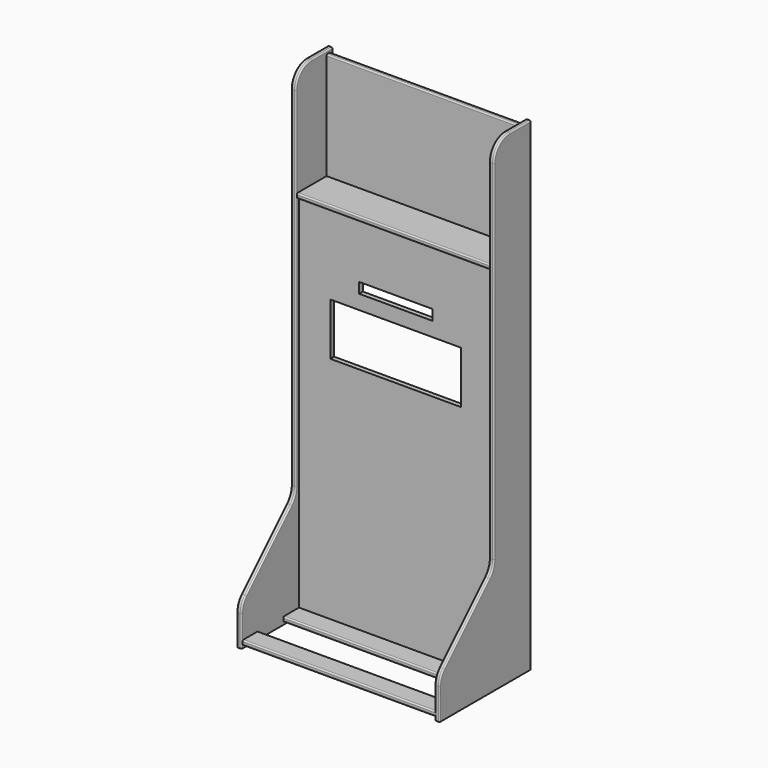
from build123d import *

# Parameters (mm, degrees)
F1_DEPTH  = 18
F3_W      = 740
F3_H      = 1382
F3_W_2    = 500
F3_H_2    = 200
F3_W_3    = 280
F3_H_3    = 40
F4_DEPTH  = 18
F7_DEPTH  = 18
F9_W      = 740
F9_H      = 160
F10_DEPTH = 18
F12_W     = 740
F12_H     = 410
F13_DEPTH = 18
F15_W     = 740
F15_H     = 225
F15_H_2   = 75
F16_DEPTH = 18
F17_R     = 4.9999


# Not quite as in the source:
# - a fillet or chamfer is up to 0.001 mm smaller than in the source, because OpenCascade refuses the exact size


with BuildPart() as f1:
    # F0 (on Right) → F1 (new body)
    with BuildSketch(Plane.YZ):
        with BuildLine():
            Line((-435, 0), (0, 0))
            Line((0, 0), (0, 1850))
            Line((0, 1850), (-100, 1850))
            ThreePointArc((-100, 1850), (-153.033008589, 1828.033008589), (-175, 1775))
            Line((-175, 1775), (-175, 441.066017178))
            ThreePointArc((-175, 441.066017178), (-180.7090350617, 412.3647597506), (-196.966991411, 388.033008589))
            Line((-196.966991411, 388.033008589), (-413.033008589, 171.966991411))
            ThreePointArc((-413.033008589, 171.966991411), (-429.2909649383, 147.6352402494), (-435, 118.933982822))
            Line((-435, 118.933982822), (-435, 0))
        make_face()
    extrude(amount=F1_DEPTH)

    # F3 (on offset) → F4 (join)
    with BuildSketch(Plane.XZ.offset(160)):
        with Locations((388, 719)):
            Rectangle(F3_W, F3_H)
        with Locations((388, 1005)):
            Rectangle(F3_W_2, F3_H_2, mode=Mode.SUBTRACT)
        with Locations((388, 1180)):
            Rectangle(F3_W_3, F3_H_3, mode=Mode.SUBTRACT)
    extrude(amount=-F4_DEPTH)

    # F6 (on offset) → F7 (join)
    with BuildSketch(Plane.YZ.offset(758)):
        with BuildLine():
            Line((-435, 0), (0, 0))
            Line((0, 0), (0, 1850))
            Line((0, 1850), (-100, 1850))
            ThreePointArc((-100, 1850), (-153.033008589, 1828.033008589), (-175, 1775))
            Line((-175, 1775), (-175, 441.066017178))
            ThreePointArc((-175, 441.066017178), (-180.7090350617, 412.3647597506), (-196.966991411, 388.033008589))
            Line((-196.966991411, 388.033008589), (-413.033008589, 171.966991411))
            ThreePointArc((-413.033008589, 171.966991411), (-429.2909649383, 147.6352402494), (-435, 118.933982822))
            Line((-435, 118.933982822), (-435, 0))
        make_face()
    extrude(amount=F7_DEPTH)

    # F9 (on offset) → F10 (join)
    with BuildSketch(Plane.XY.offset(1410)):
        with Locations((388, -90)):
            Rectangle(F9_W, F9_H)
    extrude(amount=F10_DEPTH)

    # F12 (on offset) → F13 (join)
    with BuildSketch(Plane(origin=(0, -10, 0), x_dir=(-1, 0, 0), z_dir=(0, 1, 0))):
        with Locations((-388, 1633)):
            Rectangle(F12_W, F12_H)
    extrude(amount=-F13_DEPTH)

    # F15 (on offset) → F16 (join)
    with BuildSketch(Plane(origin=(0, 0, 28), x_dir=(1, 0, 0), z_dir=(0, 0, -1))):
        with Locations((388, 122.5)):
            Rectangle(F15_W, F15_H)
        with Locations((388, 392.5)):
            Rectangle(F15_W, F15_H_2)
    extrude(amount=F16_DEPTH)

    # F17 (radius 5 in the source; OpenCascade refuses exactly that, so slightly less here)
    f17_edges = [f1.edges().sort_by_distance(p)[0] for p in [
        (388, -170, 1428),
        (388, -170, 1410),
        (758, -175, 1108.033009),
        (776, -175, 1108.033009),
        (388, -28, 1838),
        (388, -10, 1838),
        (18, -50, 1850),
        (0, -50, 1850),
        (388, -235, 28),
        (388, -355, 28),
        (388, -430, 28),
        (388, -430, 10),
        (388, -235, 10),
    ]]
    fillet(f17_edges, radius=F17_R)


solid = f1.part
